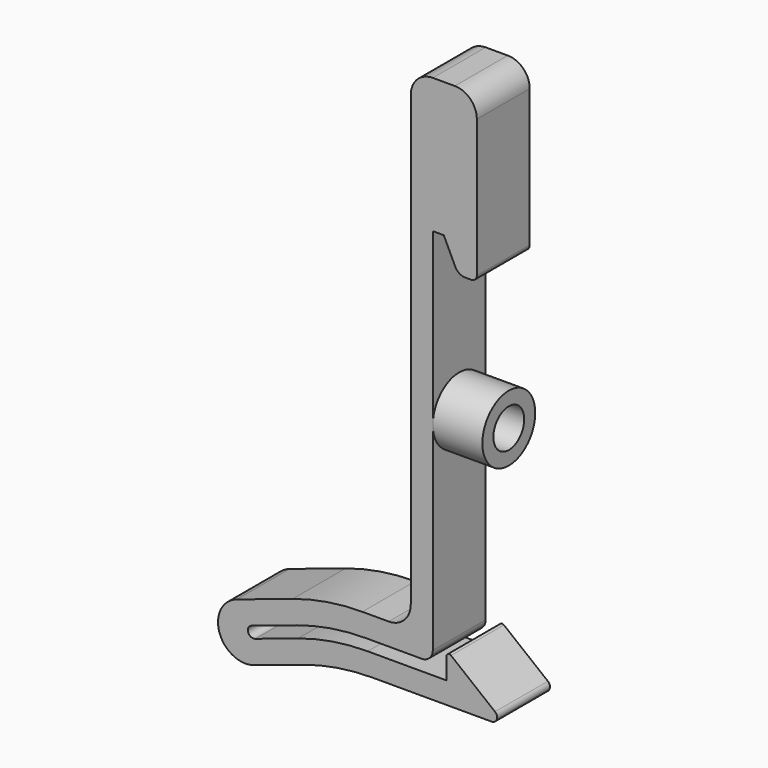
from build123d import *

# Parameters (mm, degrees)
F1_DEPTH = 6
F2_R     = 3
F3_DEPTH = 4.5
F5_D     = 3.5


# Not quite as in the source:
# - ends of sketch curves that miss each other by under 0.0002 mm in the source are joined


with BuildPart() as f1:
    # F0 (on Front) → F1 (new body)
    with BuildSketch(Plane.XZ):
        with BuildLine():
            Line((14.498358, 10), (14.498358, 14))
            Line((14.498358, 14), (14.498358, 14.25))
            Line((14.498358, 14.25), (15.498358, 14.25))
            Line((15.498358, 14.25), (16.539344, 12.069217))
            ThreePointArc((16.539344, 12.069217), (16.9083128035, 11.6541918591), (17.4418, 11.5))
            Line((17.4418, 11.5), (17.998358, 11.5))
            ThreePointArc((17.998358, 11.5), (18.3519113906, 11.6464466094), (18.498358, 12))
            Line((18.498358, 12), (18.498358, 24.5))
            ThreePointArc((18.498358, 24.5), (17.9125715624, 25.9142135624), (16.498358, 26.5))
            Line((16.498358, 26.5), (14.498358, 26.5))
            ThreePointArc((14.498358, 26.5), (13.0841444376, 25.9142135624), (12.498358, 24.5))
            Line((12.498358, 24.5), (12.498358, 22.5))
            Line((12.498358, 22.5), (12.498358, -16.25))
            ThreePointArc((12.498358, -16.25), (11.9125715624, -17.6642135624), (10.498358, -18.25))
            Line((10.498358, -18.25), (8.106805, -18.25))
            ThreePointArc((8.106805, -18.25), (4.9031601399, -18.5082508473), (1.7822496797, -19.276334039))
            Line((1.7822496797, -19.276334039), (-3.290569563, -20.9672737865))
            ThreePointArc((-3.290569563, -20.9672737865), (-4.8717084961, -24.1295514929), (-1.7094308537, -25.710690554))
            Line((-1.7094308537, -25.710690554), (2.709257, -24.237795))
            ThreePointArc((2.709257, -24.237795), (5.8301671399, -23.4697108473), (9.033812, -23.21146))
            Line((9.033812, -23.21146), (19.837293, -23.21146))
            ThreePointArc((19.837293, -23.21146), (20.3091070562, -22.8769637655), (20.1496410116, -22.3210259855))
            Line((20.1496410116, -22.3210259855), (16.154532, -19.124939))
            ThreePointArc((16.154532, -19.124939), (15.8900609581, -19.0948301233), (15.748358, -19.320156))
            Line((15.748358, -19.320156), (15.748358, -21.25))
            Line((15.748358, -21.25), (8.593639, -21.25))
            ThreePointArc((8.593639, -21.25), (5.3899932959, -21.5082508219), (2.2690829797, -22.276333939))
            Line((2.2690829797, -22.276333939), (-1.630813, -23.576299))
            ThreePointArc((-1.630813, -23.576299), (-2.263268599, -23.260072033), (-1.947040883, -22.627616351))
            Line((-1.947040883, -22.627616351), (2.106805, -21.276334))
            ThreePointArc((2.106805, -21.276334), (5.2277158277, -20.5082508979), (8.431361, -20.25))
            Line((8.431361, -20.25), (13.498358, -20.25))
            ThreePointArc((13.498358, -20.25), (14.2054647812, -19.9571067812), (14.498358, -19.25))
            Line((14.498358, -19.25), (14.498358, 10))
        make_face()
    extrude(amount=F1_DEPTH)

    # F2 (on face) → F3 (join)
    with BuildSketch(Plane.YZ.offset(14.498358)):
        with Locations((-3, -1.25)):
            Circle(F2_R)
    extrude(amount=F3_DEPTH)

    # F5 (through all)
    with Locations(Plane.YZ.offset(18.998358)):
        with Locations((-3, -1.25)):
            Hole(F5_D / 2)


solid = f1.part
